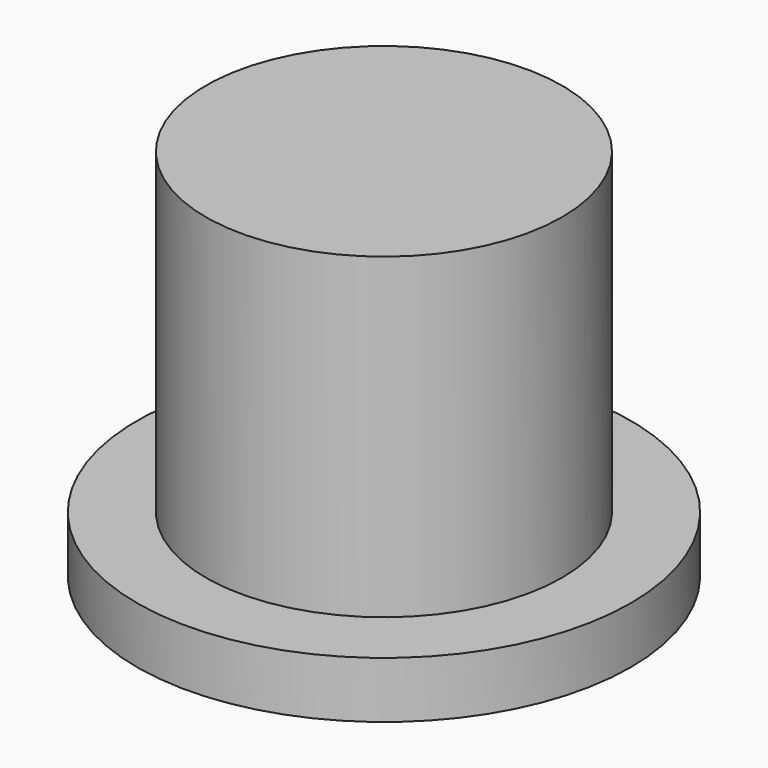
from build123d import *

# Parameters (mm, degrees)
F0_R     = 3.5
F0_R_2   = 2.525
F1_DEPTH = 0.8
F2_DEPTH = 5.3


# Not quite as in the source:
# - the program builds the solid bodies; features that only make, move or delete a surface that nothing else refers to are left out


with BuildPart() as f1:
    # F0 (on Top) → F1 (new body)
    with BuildSketch(Plane.XY):
        Circle(F0_R)
        Circle(F0_R_2, mode=Mode.SUBTRACT)
    extrude(amount=F1_DEPTH)

    # F0 (on Top) → F2 (join)
    with BuildSketch(Plane.XY):
        Circle(F0_R_2)
    extrude(amount=F2_DEPTH)


solid = f1.part
